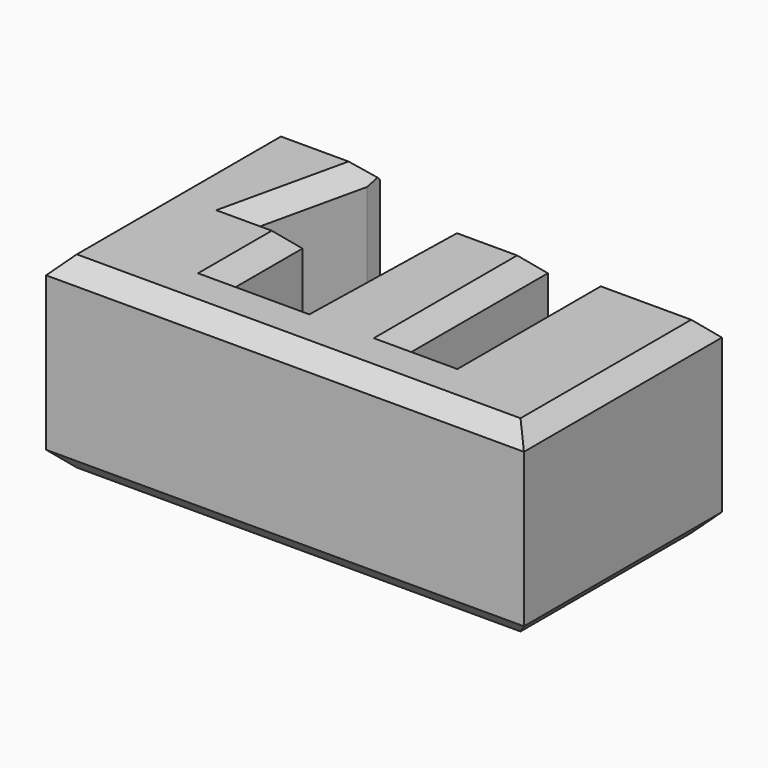
from build123d import *

# Parameters (mm, degrees)
F0_W        = 6
F0_H        = 0.95
F1_DEPTH    = 11
F2_C1_SIZE  = 1
F2_C2_SIZE  = 1
F2_C3_SIZE  = 1
F2_C4_SIZE  = 1
F2_C5_SIZE  = 1
F2_C6_SIZE  = 1
F2_C7_SIZE  = 1
F2_C8_SIZE  = 1
F2_C9_SIZE  = 1
F2_C10_SIZE = 1
F2_C11_SIZE = 1
F2_C12_SIZE = 0.9999
F2_C13_SIZE = 1
F2_C14_SIZE = 1
F3_C1_SIZE  = 1
F3_C2_SIZE  = 1
F3_C3_SIZE  = 1
F3_C4_SIZE  = 1
F3_C5_SIZE  = 1
F3_C6_SIZE  = 0.9999
F3_C7_SIZE  = 1
F3_C8_SIZE  = 1
F3_C9_SIZE  = 1
F3_C10_SIZE = 1
F3_C11_SIZE = 1
F3_C12_SIZE = 1
F3_C13_SIZE = 1
F3_C14_SIZE = 1


# Not quite as in the source:
# - a fillet or chamfer is up to 0.001 mm smaller than in the source, because OpenCascade refuses the exact size


with BuildPart() as f1:
    # F0 (on Top) → F1 (new body)
    with BuildSketch(Plane.XY):
        Polygon((0.25, 10.5), (0, 0), (-4.546, 0), (-8.77, 0), (-7.546, 5.4), (-6.05, 12), (-12.05, 12), (-12.05, -4), (15.95, -4), (15.95, 10.5), (8.65, 10.5), (8.65, 0), (5.75, 0), (5.75, 10.5), align=None)
        Polygon((-8.77, 0), (-4.546, 0), (-4.546, 5.4), (-7.546, 5.4), align=None)
        with Locations((-9.05, 12.475)):
            Rectangle(F0_W, F0_H)
    extrude(amount=F1_DEPTH)

    # F2: chamfer of 1 on 14 edges, made by hand

    # F2_c1
    f2_c1_edges = [f1.edges().sort_by_distance(p)[0] for p in [
        (0.125, 5.25, 11),
    ]]
    chamfer(f2_c1_edges, length=F2_C1_SIZE)

    # F2_c2
    f2_c2_edges = [f1.edges().sort_by_distance(p)[0] for p in [
        (-2.273, 0, 11),
    ]]
    chamfer(f2_c2_edges, length=F2_C2_SIZE)

    # F2_c3
    f2_c3_edges = [f1.edges().sort_by_distance(p)[0] for p in [
        (-4.546, 2.7, 11),
    ]]
    chamfer(f2_c3_edges, length=F2_C3_SIZE)

    # F2_c4
    f2_c4_edges = [f1.edges().sort_by_distance(p)[0] for p in [
        (-6.546, 5.4, 11),
    ]]
    chamfer(f2_c4_edges, length=F2_C4_SIZE)

    # F2_c5
    f2_c5_edges = [f1.edges().sort_by_distance(p)[0] for p in [
        (-6.798, 8.7, 11),
    ]]
    chamfer(f2_c5_edges, length=F2_C5_SIZE)

    # F2_c6
    f2_c6_edges = [f1.edges().sort_by_distance(p)[0] for p in [
        (-9.4550169048, 12.95, 11),
    ]]
    chamfer(f2_c6_edges, length=F2_C6_SIZE)

    # F2_c7
    f2_c7_edges = [f1.edges().sort_by_distance(p)[0] for p in [
        (-12.05, 3.975, 11),
    ]]
    chamfer(f2_c7_edges, length=F2_C7_SIZE)

    # F2_c8
    f2_c8_edges = [f1.edges().sort_by_distance(p)[0] for p in [
        (2.45, -4, 11),
    ]]
    chamfer(f2_c8_edges, length=F2_C8_SIZE)

    # F2_c9
    f2_c9_edges = [f1.edges().sort_by_distance(p)[0] for p in [
        (15.95, 3.75, 11),
    ]]
    chamfer(f2_c9_edges, length=F2_C9_SIZE)

    # F2_c10
    f2_c10_edges = [f1.edges().sort_by_distance(p)[0] for p in [
        (11.8, 10.5, 11),
    ]]
    chamfer(f2_c10_edges, length=F2_C10_SIZE)

    # F2_c11
    f2_c11_edges = [f1.edges().sort_by_distance(p)[0] for p in [
        (8.65, 4.75, 11),
    ]]
    chamfer(f2_c11_edges, length=F2_C11_SIZE)

    # F2_c12 (size 1 in the source; OpenCascade refuses exactly that, so slightly less here)
    f2_c12_edges = [f1.edges().sort_by_distance(p)[0] for p in [
        (7.2, 0, 11),
    ]]
    chamfer(f2_c12_edges, length=F2_C12_SIZE)

    # F2_c13
    f2_c13_edges = [f1.edges().sort_by_distance(p)[0] for p in [
        (5.75, 5.25, 11),
    ]]
    chamfer(f2_c13_edges, length=F2_C13_SIZE)

    # F2_c14
    f2_c14_edges = [f1.edges().sort_by_distance(p)[0] for p in [
        (3.0001417033, 10.5, 11),
    ]]
    chamfer(f2_c14_edges, length=F2_C14_SIZE)

    # F3: chamfer of 1 on 14 edges, made by hand

    # F3_c1
    f3_c1_edges = [f1.edges().sort_by_distance(p)[0] for p in [
        (5.75, 5.25, 0),
    ]]
    chamfer(f3_c1_edges, length=F3_C1_SIZE)

    # F3_c2
    f3_c2_edges = [f1.edges().sort_by_distance(p)[0] for p in [
        (7.2, 0, 0),
    ]]
    chamfer(f3_c2_edges, length=F3_C2_SIZE)

    # F3_c3
    f3_c3_edges = [f1.edges().sort_by_distance(p)[0] for p in [
        (2.5, 10.5, 0),
    ]]
    chamfer(f3_c3_edges, length=F3_C3_SIZE)

    # F3_c4
    f3_c4_edges = [f1.edges().sort_by_distance(p)[0] for p in [
        (0.1130952381, 4.75, 0),
    ]]
    chamfer(f3_c4_edges, length=F3_C4_SIZE)

    # F3_c5
    f3_c5_edges = [f1.edges().sort_by_distance(p)[0] for p in [
        (8.65, 5.25, 0),
    ]]
    chamfer(f3_c5_edges, length=F3_C5_SIZE)

    # F3_c6 (size 1 in the source; OpenCascade refuses exactly that, so slightly less here)
    f3_c6_edges = [f1.edges().sort_by_distance(p)[0] for p in [
        (-2.273, 0, 0),
    ]]
    chamfer(f3_c6_edges, length=F3_C6_SIZE)

    # F3_c7
    f3_c7_edges = [f1.edges().sort_by_distance(p)[0] for p in [
        (12.8, 10.5, 0),
    ]]
    chamfer(f3_c7_edges, length=F3_C7_SIZE)

    # F3_c8
    f3_c8_edges = [f1.edges().sort_by_distance(p)[0] for p in [
        (15.95, 2.75, 0),
    ]]
    chamfer(f3_c8_edges, length=F3_C8_SIZE)

    # F3_c9
    f3_c9_edges = [f1.edges().sort_by_distance(p)[0] for p in [
        (-4.546, 2.7, 0),
    ]]
    chamfer(f3_c9_edges, length=F3_C9_SIZE)

    # F3_c10
    f3_c10_edges = [f1.edges().sort_by_distance(p)[0] for p in [
        (1.45, -4, 0),
    ]]
    chamfer(f3_c10_edges, length=F3_C10_SIZE)

    # F3_c11
    f3_c11_edges = [f1.edges().sort_by_distance(p)[0] for p in [
        (-6.546, 5.4, 0),
    ]]
    chamfer(f3_c11_edges, length=F3_C11_SIZE)

    # F3_c12
    f3_c12_edges = [f1.edges().sort_by_distance(p)[0] for p in [
        (-12.05, 4.975, 0),
    ]]
    chamfer(f3_c12_edges, length=F3_C12_SIZE)

    # F3_c13
    f3_c13_edges = [f1.edges().sort_by_distance(p)[0] for p in [
        (-8.55, 12.95, 0),
    ]]
    chamfer(f3_c13_edges, length=F3_C13_SIZE)

    # F3_c14
    f3_c14_edges = [f1.edges().sort_by_distance(p)[0] for p in [
        (-6.8036666667, 8.675, 0),
    ]]
    chamfer(f3_c14_edges, length=F3_C14_SIZE)


solid = f1.part
